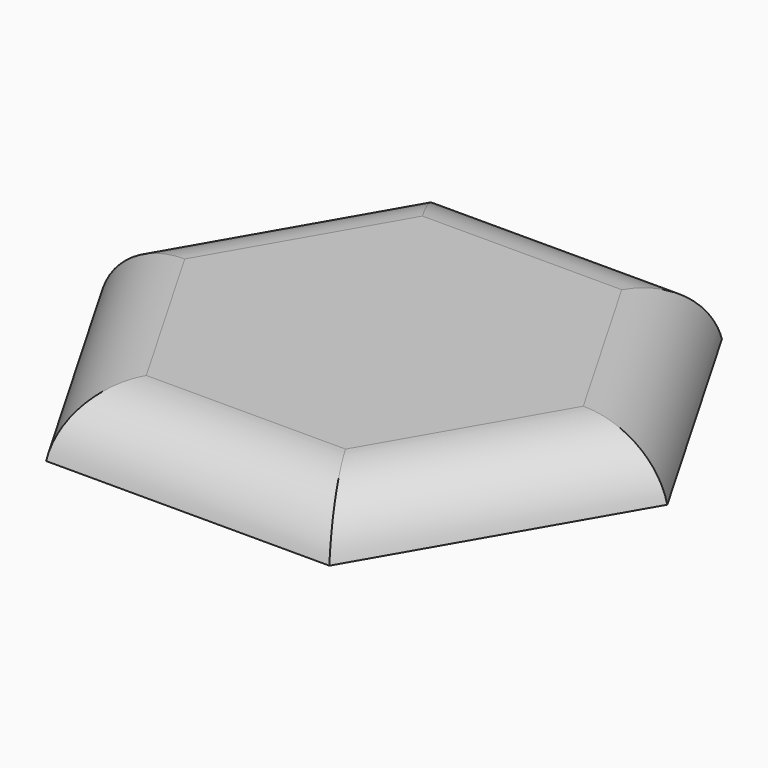
from build123d import *

# Parameters (mm, degrees)
F1_DEPTH    = 4
F2_T1_DEPTH = 43.5711374279
F2_T3_DEPTH = 43.5711374279
F2_T5_DEPTH = 43.5711374279
F2_T7_DEPTH = 43.5711374279
F2_T9_DEPTH = 43.5711374279


# Not quite as in the source:
# - a fillet or chamfer that OpenCascade refuses, or shapes differently, is made with other operations: its cross-section is extruded or revolved along the edge and cut away or added


with BuildPart() as f1:
    # F0 (on Top) → F1 (new body)
    with BuildSketch(Plane.XY):
        Polygon((-9.53812, 16.5205084487), (0, 0), (9.53812, 16.5205084487), align=None)
        Polygon((-19.07624, 0), (0, 0), (-9.53812, 16.5205084487), align=None)
        Polygon((-9.53812, -16.5205084487), (0, 0), (-19.07624, 0), align=None)
        Polygon((9.53812, -16.5205084487), (0, 0), (-9.53812, -16.5205084487), align=None)
        Polygon((19.07624, 0), (0, 0), (9.53812, -16.5205084487), align=None)
        Polygon((9.53812, 16.5205084487), (0, 0), (19.07624, 0), align=None)
    extrude(amount=F1_DEPTH)

    # F2: fillet of radius 5 on 6 edges, made by hand

    # F2_s2 → F2_t1 (cut)
    with BuildSketch(Plane.YZ.offset(-21.7855687139)):
        with BuildLine():
            ThreePointArc((16.5205084487, 0), (14.7838066233, 2.8729833462), (11.6215289631, 4))
            Line((11.6215289631, 4), (16.5205084487, 4))
            Line((16.5205084487, 4), (16.5205084487, 0))
        make_face()
        with BuildLine():
            ThreePointArc((-16.5205084487, 0), (-14.7838066233, 2.8729833462), (-11.6215289631, 4))
            Line((-11.6215289631, 4), (-16.5205084487, 4))
            Line((-16.5205084487, 4), (-16.5205084487, 0))
        make_face()
    extrude(amount=F2_T1_DEPTH, mode=Mode.SUBTRACT)

    # F2_s4 → F2_t3 (cut)
    with BuildSketch(Plane(origin=(10.892784357, 18.8668559422, 0), x_dir=(0, 0, 1), z_dir=(-0.5, -0.8660254038, 0))):
        with BuildLine():
            ThreePointArc((0, 16.5205084487), (2.8729833462, 14.7838066233), (4, 11.6215289631))
            Line((4, 11.6215289631), (4, 16.5205084487))
            Line((4, 16.5205084487), (0, 16.5205084487))
        make_face()
    extrude(amount=F2_T3_DEPTH, mode=Mode.SUBTRACT)

    # F2_s6 → F2_t5 (cut)
    with BuildSketch(Plane(origin=(-10.892784357, 18.8668559422, 0), x_dir=(0, 0, 1), z_dir=(0.5, -0.8660254038, 0))):
        with BuildLine():
            ThreePointArc((0, 16.5205084487), (2.8729833462, 14.7838066233), (4, 11.6215289631))
            Line((4, 11.6215289631), (4, 16.5205084487))
            Line((4, 16.5205084487), (0, 16.5205084487))
        make_face()
    extrude(amount=F2_T5_DEPTH, mode=Mode.SUBTRACT)

    # F2_s8 → F2_t7 (cut)
    with BuildSketch(Plane(origin=(10.892784357, -18.8668559422, 0), x_dir=(0, 0, 1), z_dir=(-0.5, 0.8660254038, 0))):
        with BuildLine():
            ThreePointArc((0, 16.5205084487), (2.8729833462, 14.7838066233), (4, 11.6215289631))
            Line((4, 11.6215289631), (4, 16.5205084487))
            Line((4, 16.5205084487), (0, 16.5205084487))
        make_face()
    extrude(amount=F2_T7_DEPTH, mode=Mode.SUBTRACT)

    # F2_s10 → F2_t9 (cut)
    with BuildSketch(Plane(origin=(-10.892784357, -18.8668559422, 0), x_dir=(0, 0, 1), z_dir=(0.5, 0.8660254038, 0))):
        with BuildLine():
            ThreePointArc((0, 16.5205084487), (2.8729833462, 14.7838066233), (4, 11.6215289631))
            Line((4, 11.6215289631), (4, 16.5205084487))
            Line((4, 16.5205084487), (0, 16.5205084487))
        make_face()
    extrude(amount=F2_T9_DEPTH, mode=Mode.SUBTRACT)


solid = f1.part
